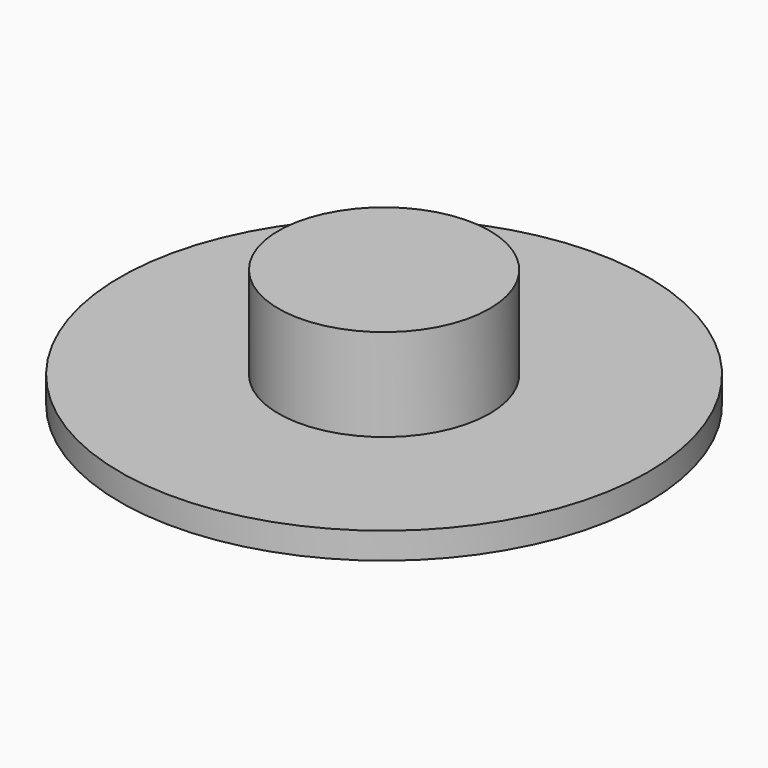
from build123d import *

# Parameters (mm, degrees)
F0_R         = 10
F1_DEPTH     = 1
F2_R         = 4
F3_DEPTH     = 3.5
F4_TEXT_SIZE = 9.2307692308
F5_DEPTH     = 0.5


# Not quite as in the source:
# - Text() gives the source's letters only with a copy of the font that has no kerning and outlines rounded to 1/6400 em; it was checked with that copy


with BuildPart() as f1:
    # F0 (on Top) → F1 (new body)
    with BuildSketch(Plane.XY):
        Circle(F0_R)
    extrude(amount=F1_DEPTH)

    # F2 (on face) → F3 (join)
    with BuildSketch(Plane.XY.offset(1)):
        Circle(F2_R)
    extrude(amount=F3_DEPTH)

    # F4 (on face) → F5 (join)
    with BuildSketch(Plane(origin=(0, 0, 0), x_dir=(1, 0, 0), z_dir=(0, 0, -1))):
        with Locations((-7.34771841, -3.4620246111)):
            Text('BW', F4_TEXT_SIZE, font='Open Sans', text_align=(TextAlign.LEFT, TextAlign.BOTTOM))
    extrude(amount=F5_DEPTH)


solid = f1.part
